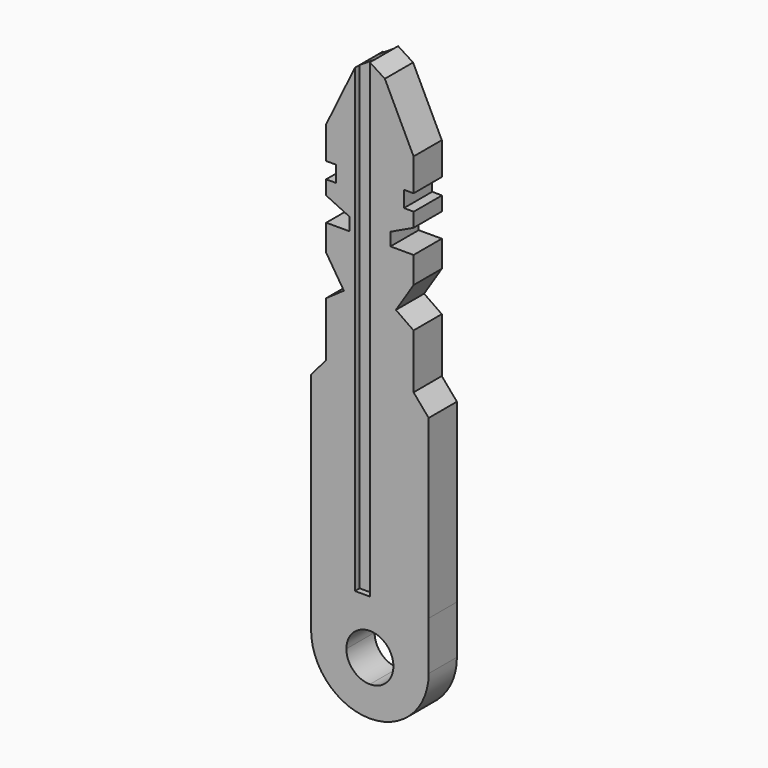
from build123d import *

# Parameters (mm, degrees)
F1_DEPTH = 1.5
F3_DEPTH = 0.5
F5_DEPTH = 0.5
F7_DEPTH = 3


# Not quite as in the source:
# - ends of sketch curves that miss each other by under 0.0002 mm in the source are joined
# - a feature names something its author has since deleted; it is built from what else it names


with BuildPart() as f1:
    # F0 (on Front) → F1 (new body, symmetric)
    with BuildSketch(Plane.XZ):
        Polygon((0, 40), (0, 0), (5, 0), (5, 15), (3.7145695426, 16.5003631264), (3.7145695426, 21.137110889), (2.2125243451, 22.1820119768), (3.7145695426, 24.5330389589), (3.7145695426, 26.7870686948), (1.7496975381, 26.7870686948), (1.7496975381, 27.8878770769), (3.7145695426, 28.8214460015), (3.7266683541, 30.0295948982), (2.903013601, 30.0378432554), (2.903013601, 31.4024910331), (3.7145695426, 31.4024910331), (3.7145695426, 34.1644659638), (1.2732772157, 39.1865172364), align=None)
        Polygon((-1.2732772157, 0), (0, 0), (0, 40), (-1.2732772157, 39.1865172364), align=None)
        Polygon((-5, 0), (-1.2732772157, 0), (-1.2732772157, 39.1865172364), (-3.7145695426, 34.1644659638), (-3.7145695426, 31.4024910331), (-2.903013601, 31.4024910331), (-2.903013601, 30.0378432554), (-3.7266683541, 30.0295948982), (-3.7145695426, 28.8214460015), (-1.7496975381, 27.8878770769), (-1.7496975381, 26.7870686948), (-3.7145695426, 26.7870686948), (-3.7145695426, 24.5330389589), (-2.2125243451, 22.1820119768), (-3.7145695426, 21.137110889), (-3.7145695426, 16.5003631264), (-5, 15), align=None)
    extrude(amount=F1_DEPTH, both=True)

    # F2 (on face) → F3 (cut)
    with BuildSketch(Plane.XZ.offset(1.5)):
        Polygon((0, 0), (0, 40), (-1.2732772157, 39.1865172364), (-1.2732772157, 0), align=None)
    extrude(amount=-F3_DEPTH, mode=Mode.SUBTRACT)

    # F4 (on face) → F5 (cut)
    with BuildSketch(Plane(origin=(0, 1.5, 0), x_dir=(-1, 0, 0), z_dir=(0, 1, 0))):
        Polygon((1.2732772157, 0), (1.2732772157, 39.1865172364), (0, 40), (0, 0), align=None)
    extrude(amount=-F5_DEPTH, mode=Mode.SUBTRACT)

    # F6 (on face) → F7 (join)
    with BuildSketch(Plane(origin=(0, 1.5, 0), x_dir=(-1, 0, 0), z_dir=(0, 1, 0))):
        with BuildLine():
            Line((-5, 0), (-4.9999982459, -4.1340150831))
            ThreePointArc((-4.9999982459, -4.1340150831), (-3.5355314017, -7.6695476176), (1.7541e-06, -9.1340129616))
            Line((1.7541e-06, -9.1340129616), (1.3932e-06, -6.5670064808))
            ThreePointArc((1.3932e-06, -6.5670064808), (-1.9999990311, -4.5670062085), (5.446e-07, -2.5670064808))
            Line((5.446e-07, -2.5670064808), (0, 0))
            Line((0, 0), (-5, 0))
        make_face()
        with BuildLine():
            Line((1.3932e-06, -6.5670064808), (1.9378e-06, -9.1340129616))
            ThreePointArc((1.9378e-06, -9.1340129616), (3.5355339059, -7.6695468675), (5, -4.1340129616))
            Line((5, -4.1340129616), (5, 0))
            Line((5, 0), (0, 0))
            Line((0, 0), (5.446e-07, -2.5670064808))
            ThreePointArc((5.446e-07, -2.5670064808), (1.4142143813, -3.1527927684), (2.0000009689, -4.5670064808))
            ThreePointArc((2.0000009689, -4.5670064808), (1.4142141887, -5.9812203857), (1.3932e-06, -6.5670064808))
        make_face()
    extrude(amount=-F7_DEPTH)


solid = f1.part
